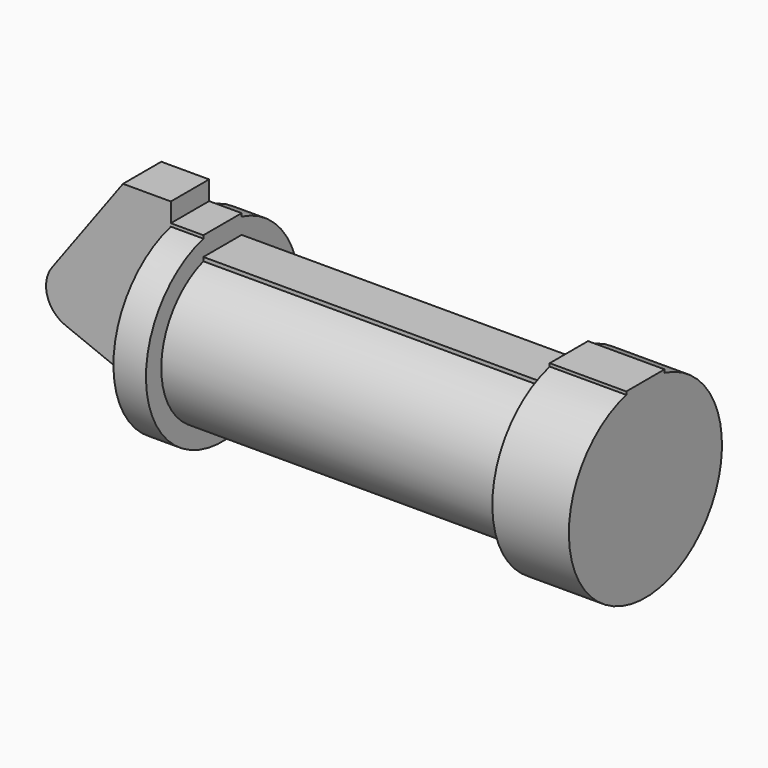
from build123d import *

# Parameters (mm, degrees)
F0_W     = 5.842
F0_H     = 12.7
F0_R     = 1.524
F2_DEPTH = 3.175


with BuildPart() as f1:
    # F0 (on Front) → F1 (revolve)
    with BuildSketch(Plane.XZ):
        Polygon((5.842, 12.7), (5.842, 0), (66.294, 0), (66.294, 12.7), (56.134, 12.7), (56.134, 10.16), (10.16, 10.16), (10.16, 12.7), align=None)
    revolve(axis=Axis((33.147, 0, 0), (-1, 0, 0)))

    # F0 (on Front) → F2 (join, symmetric)
    with BuildSketch(Plane.XZ):
        Polygon((5.842, 12.7), (5.842, 0), (66.294, 0), (66.294, 12.7), (56.134, 12.7), (56.134, 10.16), (10.16, 10.16), (10.16, 12.7), align=None)
        with BuildLine():
            Line((-2.5908, 0), (0, 0))
            Line((0, 0), (0, 12.7))
            Line((0, 12.7), (5.842, 12.7))
            Line((5.842, 12.7), (5.842, 15.24))
            Line((5.842, 15.24), (-0.508, 15.24))
            Line((-0.508, 15.24), (-9.9307574264, 2.405036162))
            ThreePointArc((-9.9307574264, 2.405036162), (-5.3893741786, 3.8619675672), (-2.5908, 0))
        make_face()
        with Locations((2.921, 6.35)):
            Rectangle(F0_W, F0_H)
        with BuildLine():
            Line((5.842, 0), (0, 0))
            Line((0, 0), (-2.5908, 0))
            ThreePointArc((-2.5908, 0), (-4.3787043805, -3.3668211611), (-8.1692865802, -3.7712632364))
            Line((-8.1692865802, -3.7712632364), (5.842, -9.398))
            Line((5.842, -9.398), (5.842, 0))
        make_face()
        with BuildLine():
            ThreePointArc((-8.1692865802, -3.7712632364), (-4.3787043805, -3.3668211611), (-2.5908, 0))
            ThreePointArc((-2.5908, 0), (-5.3893741786, 3.8619675672), (-9.9307574264, 2.405036162))
            ThreePointArc((-9.9307574264, 2.405036162), (-10.5629654276, -1.1146026154), (-8.1692865802, -3.7712632364))
        make_face()
        with Locations((-6.6548, 0)):
            Circle(F0_R, mode=Mode.SUBTRACT)
        with Locations((-6.6548, 0)):
            Circle(F0_R)
    extrude(amount=F2_DEPTH, both=True)


solid = f1.part
